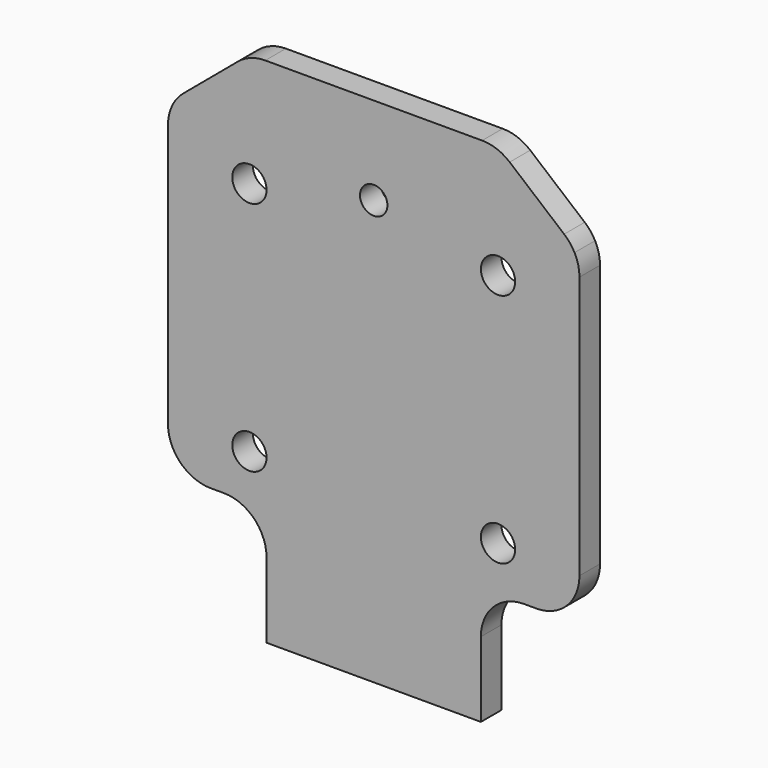
from build123d import *

# Parameters (mm, degrees)
F0_R     = 2
F0_R_2   = 1.6
F1_DEPTH = 3


# Not quite as in the source:
# - a feature names something its author has since deleted; it is built from what else it names


with BuildPart() as f1:
    # F0 (on Front) → F1 (new body)
    with BuildSketch(Plane.XZ):
        with BuildLine():
            ThreePointArc((1.7860619516, 39.4986839248), (1.1086440911, 38.8081032796), (0.5768869335, 38))
            Line((0.5768869335, 38), (47.4231130665, 38))
            ThreePointArc((47.4231130665, 38), (46.8913559089, 38.8081032796), (46.2139380484, 39.4986839248))
            Line((46.2139380484, 39.4986839248), (39.8600581363, 44.8302222156))
            ThreePointArc((39.8600581363, 44.8302222156), (38.3562208045, 45.6984631039), (36.6461200879, 46))
            Line((36.6461200879, 46), (11.3538799121, 46))
            ThreePointArc((11.3538799121, 46), (9.6437791955, 45.6984631039), (8.1399418637, 44.8302222156))
            Line((8.1399418637, 44.8302222156), (1.7860619516, 39.4986839248))
        make_face()
        with BuildLine():
            Line((47.4231130665, 38), (0.5768869335, 38))
            ThreePointArc((0.5768869335, 38), (0.1463639747, 36.869385243), (0, 35.6684617092))
            Line((0, 35.6684617092), (0, 5))
            ThreePointArc((0, 5), (1.4644660941, 1.4644660941), (5, 0))
            Line((5, 0), (6.5, 0))
            ThreePointArc((6.5, 0), (10.0355339059, -1.4644660941), (11.5, -5))
            Line((11.5, -5), (11.5, -5.0126606831))
            Line((11.5, -5.0126606831), (11.5, -13.75))
            Line((11.5, -13.75), (36.5, -13.75))
            Line((36.5, -13.75), (36.5, -5))
            ThreePointArc((36.5, -5), (37.9644660941, -1.4644660941), (41.5, 0))
            Line((41.5, 0), (43, 0))
            ThreePointArc((43, 0), (46.5355339059, 1.4644660941), (48, 5))
            Line((48, 5), (48, 35.6684617092))
            ThreePointArc((48, 35.6684617092), (47.8536360253, 36.869385243), (47.4231130665, 38))
        make_face()
        with Locations((9.5, 5.25)):
            Circle(F0_R, mode=Mode.SUBTRACT)
        with Locations((38.5, 5.25)):
            Circle(F0_R, mode=Mode.SUBTRACT)
        with Locations((9.5, 32.75)):
            Circle(F0_R, mode=Mode.SUBTRACT)
        with Locations((24, 35.75)):
            Circle(F0_R_2, mode=Mode.SUBTRACT)
        with Locations((38.5, 32.75)):
            Circle(F0_R, mode=Mode.SUBTRACT)
    extrude(amount=F1_DEPTH)


solid = f1.part
